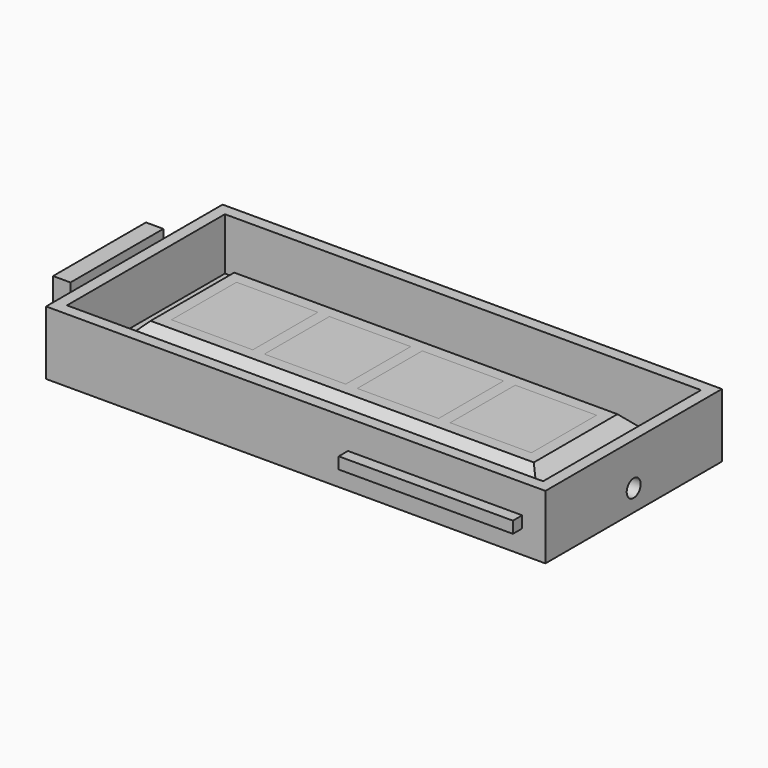
from build123d import *

# Parameters (mm, degrees)
F2_W      = 33
F2_H      = 9
F0_W      = 39
F0_H      = 15
F4_W      = 7
F4_H      = 7
F5_DEPTH  = 0.5
F6_DEPTH  = 0.5
F7_W      = 43
F7_H      = 19
F7_W_2    = 41
F7_H_2    = 17
F7_W_3    = 39
F7_H_3    = 15
F8_DEPTH  = 1
F9_DEPTH  = 4.5
F10_R     = 0.75
F11_DEPTH = 1
F12_W     = 15
F12_H     = 1
F13_DEPTH = 1
F18_DEPTH = 5


# Not quite as in the source:
# - a feature of the source that left no trace in its solid (it failed there, or was rolled back) is left out
# - a pattern or mirror of a feature is missing from the dataset's text; its kind, count and spacing are read off the source's solid


with BuildPart() as f3:
    # F2 (on offset) → F3 section 0
    with BuildSketch(Plane.XY.offset(3)):
        with Locations((16.5, 4.5)):
            Rectangle(F2_W, F2_H)
    # F0 (on Top) → F3 section 1
    with BuildSketch(Plane.XY):
        with Locations((16.5, 4.5)):
            Rectangle(F0_W, F0_H)
    loft()

    # F4 (on offset) → F5 (cut)
    with BuildSketch(Plane.XY.offset(3)):
        with Locations((28.5, 4.5)):
            Rectangle(F4_W, F4_H)
        with Locations((20.5, 4.5)):
            Rectangle(F4_W, F4_H)
        with Locations((12.5, 4.5)):
            Rectangle(F4_W, F4_H)
        with Locations((4.5, 4.5)):
            Rectangle(F4_W, F4_H)
    extrude(amount=-F5_DEPTH, mode=Mode.SUBTRACT)

    # F7 (on face) → F8 (join)
    with BuildSketch(Plane(origin=(0, 0, 0), x_dir=(1, 0, 0), z_dir=(0, 0, -1))):
        with Locations((16.5, -4.5)):
            Rectangle(F7_W, F7_H)
        with Locations((16.5, -4.5)):
            Rectangle(F7_W_2, F7_H_2, mode=Mode.SUBTRACT)
        with Locations((16.5, -4.5)):
            Rectangle(F7_W_2, F7_H_2)
        with Locations((16.5, -4.5)):
            Rectangle(F7_W_3, F7_H_3, mode=Mode.SUBTRACT)
        with Locations((16.5, -4.5)):
            Rectangle(F7_W_3, F7_H_3)
    extrude(amount=F8_DEPTH)

    # F7 (on face) → F9 (join)
    with BuildSketch(Plane(origin=(0, 0, 0), x_dir=(1, 0, 0), z_dir=(0, 0, -1))):
        with Locations((16.5, -4.5)):
            Rectangle(F7_W, F7_H)
        with Locations((16.5, -4.5)):
            Rectangle(F7_W_2, F7_H_2, mode=Mode.SUBTRACT)
    extrude(amount=-F9_DEPTH)

    # F10 (on face) → F11 (cut, through all)
    with BuildSketch(Plane.YZ.offset(38)):
        with Locations((4.5, 0.85)):
            Circle(F10_R)
    extrude(amount=-F11_DEPTH, mode=Mode.SUBTRACT)

    # F12 (on face) → F13 (join)
    with BuildSketch(Plane.XZ.offset(5)):
        with Locations((28.5, 1.5)):
            Rectangle(F12_W, F12_H)
    f13 = extrude(amount=F13_DEPTH)

    # F13_copies: F13 across plane
    add(f13.mirror(Plane.ZX.offset(4.5)))

    # F17 (on face) → F18 (join, symmetric)
    with BuildSketch(Plane(origin=(0, 4.5, 0), x_dir=(-1, 0, 0), z_dir=(0, 1, 0))):
        Polygon((6.5, 1.75), (6.5, 1), (6.5, -0.5), (8, -0.5), (8, 4), (6.5, 4), (6.5, 2.5), align=None)
        Polygon((5, 2.5), (5, 1), (6.5, 1), (6.5, 1.75), (6.5, 2.5), align=None)
    extrude(amount=F18_DEPTH, both=True)


with BuildPart() as f6:
    # F4 (on offset) → F6 (new body)
    with BuildSketch(Plane.XY.offset(3)):
        with Locations((4.5, 4.5)):
            Rectangle(F4_W, F4_H)
    extrude(amount=-F6_DEPTH)


with BuildPart() as f6b:
    # F4 (on offset) → F6, piece 2 (new body)
    with BuildSketch(Plane.XY.offset(3)):
        with Locations((12.5, 4.5)):
            Rectangle(F4_W, F4_H)
    extrude(amount=-F6_DEPTH)


with BuildPart() as f6c:
    # F4 (on offset) → F6, piece 3 (new body)
    with BuildSketch(Plane.XY.offset(3)):
        with Locations((20.5, 4.5)):
            Rectangle(F4_W, F4_H)
    extrude(amount=-F6_DEPTH)


with BuildPart() as f6d:
    # F4 (on offset) → F6, piece 4 (new body)
    with BuildSketch(Plane.XY.offset(3)):
        with Locations((28.5, 4.5)):
            Rectangle(F4_W, F4_H)
    extrude(amount=-F6_DEPTH)


solid = Compound([f3.part, f6.part, f6b.part, f6c.part, f6d.part])
